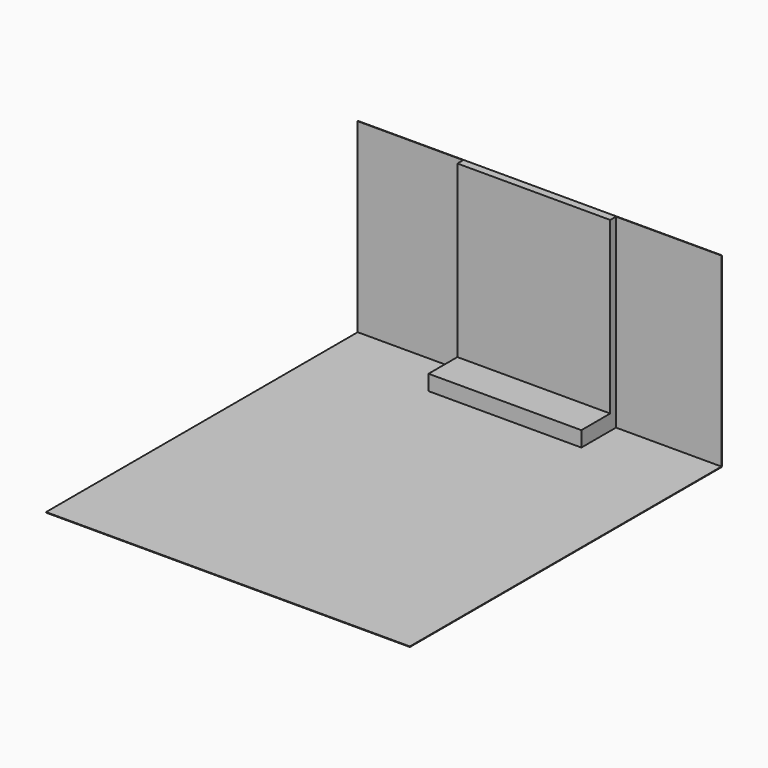
from build123d import *

# Parameters (mm, degrees)
F1_DEPTH = 5486.4
F0_W     = 1076.325
F0_H     = 215.9
F2_DEPTH = 609.6
F3_DEPTH = 101.6
F5_DEPTH = 7.9375


# Not quite as in the source:
# - a length typed as a fraction of an inch, garbled in the dataset ("3 / 203.2 mm" for 3/8 in), is restored


with BuildPart() as f1:
    # F0 (on Front) → F1 (new body)
    with BuildSketch(Plane.XZ):
        Polygon((-2562.225, 0), (-2562.225, -7.9375), (2562.225, -7.9375), (2562.225, 0), (1076.325, 0), (0, 0), (-1076.325, 0), align=None)
    extrude(amount=F1_DEPTH)


with BuildPart() as f2:
    # F0 (on Front) → F2 (new body)
    with BuildSketch(Plane.XZ):
        with Locations((538.1625, 107.95)):
            Rectangle(F0_W, F0_H)
        with Locations((-538.1625, 107.95)):
            Rectangle(F0_W, F0_H)
    extrude(amount=F2_DEPTH)

    # F0 (on Front) → F3 (join)
    with BuildSketch(Plane.XZ):
        Polygon((-1076.325, 2616.2), (-1076.325, 215.9), (0, 215.9), (1076.325, 215.9), (1076.325, 2616.2), align=None)
    extrude(amount=F3_DEPTH)


with BuildPart() as f5:
    # F4 (on Front) → F5 (new body)
    with BuildSketch(Plane.XZ):
        Polygon((-2562.225, 2616.2), (-2562.225, 0), (2562.225, 0), (2562.225, 2616.2), (1076.325, 2616.2), (-1076.325, 2616.2), align=None)
    extrude(amount=-F5_DEPTH)


solid = Compound([f1.part, f2.part, f5.part])
